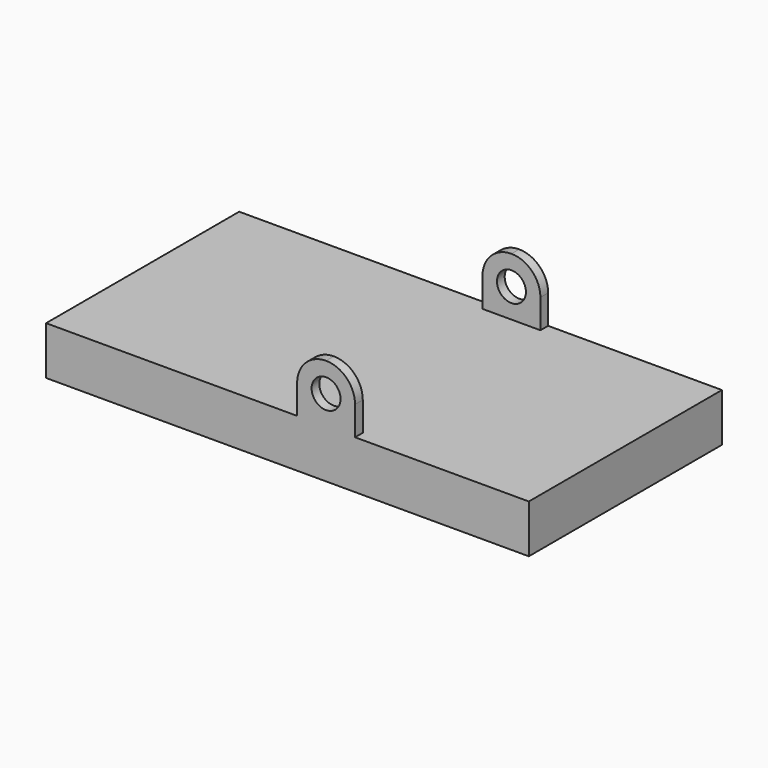
from build123d import *

# Parameters (mm, degrees)
F0_W      = 40
F0_H      = 25
F1_DEPTH  = 5
F4_W      = 6
F4_H      = 6
F5_DEPTH  = 1
F3_W      = 6
F3_H      = 6
F6_DEPTH  = 1
F7_R      = 2.99999
F8_R      = 1.5
F9_DEPTH  = 30
F10_DEPTH = 10


# Not quite as in the source:
# - a fillet or chamfer is up to 0.001 mm smaller than in the source, because OpenCascade refuses the exact size


with BuildPart() as f1:
    # F0 (on Top) → F1 (new body)
    with BuildSketch(Plane.XY):
        Rectangle(F0_W, F0_H)
    extrude(amount=F1_DEPTH)

    # F4 (on face) → F5 (join)
    with BuildSketch(Plane.XZ.offset(12.5)):
        with Locations((9, 8)):
            Rectangle(F4_W, F4_H)
    extrude(amount=-F5_DEPTH)

    # F3 (on face) → F6 (join)
    with BuildSketch(Plane(origin=(0, 12.5, 0), x_dir=(-1, 0, 0), z_dir=(0, 1, 0))):
        with Locations((-9, 8)):
            Rectangle(F3_W, F3_H)
    extrude(amount=-F6_DEPTH)

    # F7 (radius 3 in the source; OpenCascade refuses exactly that, so slightly less here)
    f7_edges = [f1.edges().sort_by_distance(p)[0] for p in [
        (6, 12, 11),
        (12, 12, 11),
        (6, -12, 11),
        (12, -12, 11),
    ]]
    fillet(f7_edges, radius=F7_R)

    # F8 (on face) → F9 (cut)
    with BuildSketch(Plane(origin=(0, 12.5, 0), x_dir=(-1, 0, 0), z_dir=(0, 1, 0))):
        with Locations((-9, 8)):
            Circle(F8_R)
    extrude(amount=-F9_DEPTH, mode=Mode.SUBTRACT)

    # F10 (add): a face of the model
    f10_faces = [f1.faces().sort_by_distance(p)[0] for p in [
        (20, 0, 2.5),
    ]]
    extrude(f10_faces, amount=F10_DEPTH)


solid = f1.part
